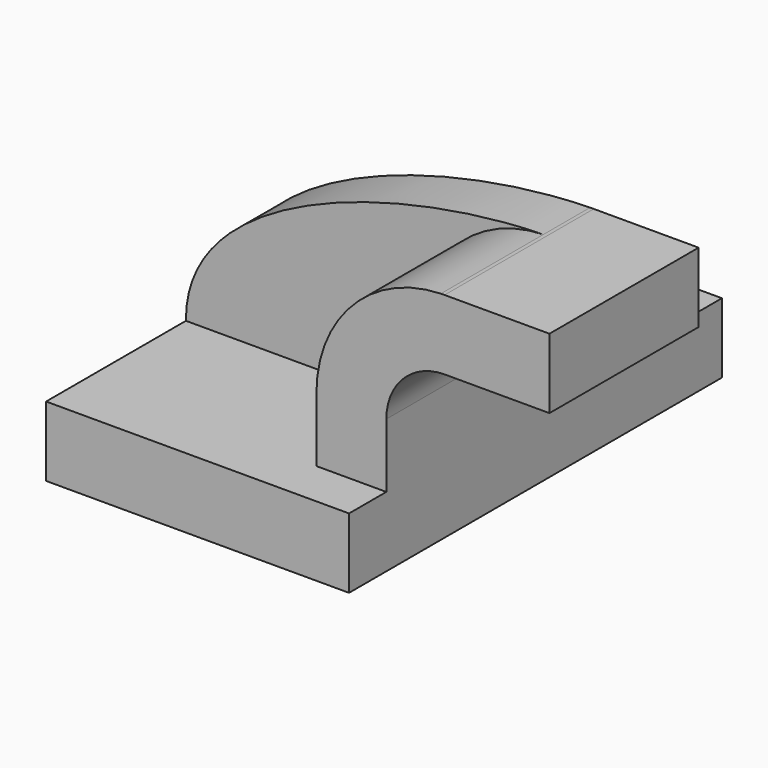
from build123d import *

# Parameters (mm, degrees)
F1_DEPTH = 63.5
F0_W     = 25.4
F0_H     = 19.0500033191
F2_DEPTH = 50.8
F3_DEPTH = 15.875


# Not quite as in the source:
# - ends of sketch curves that miss each other by under 0.0002 mm in the source are joined


with BuildPart() as f1:
    # F0 (on Front) → F1 (new body, symmetric)
    with BuildSketch(Plane.XZ):
        Polygon((-41.275, 9.525), (-41.275, -9.525), (41.275, -9.525), (41.275, 9.525), (22.225, 9.525), align=None)
    extrude(amount=F1_DEPTH, both=True)

    # F0 (on Front) → F2 (join)
    with BuildSketch(Plane.XZ):
        with BuildLine():
            Line((22.225, 9.525), (41.275, 9.525))
            Line((41.275, 9.525), (41.275, 27.0002))
            ThreePointArc((41.275, 27.0002), (45.9246798487, 38.2255201513), (57.15, 42.8752))
            Line((57.15, 42.8752), (60.325, 42.8751966809))
            Line((60.325, 42.8751966809), (60.325, 61.9252))
            Line((60.325, 61.9252), (57.15, 61.9252))
            add(Edge.make_bspline(
                [(56.1392549791, 61.9105712312), (56.4777228602, 61.916713038), (56.8146554612, 61.9215892093), (57.15, 61.9252)],
                knots=[110.5401994714, 110.5401994714, 110.5401994714, 110.5401994714, 111.5045361635, 111.5045361635, 111.5045361635, 111.5045361635], degree=3))
            ThreePointArc((56.1392549791, 61.9105712312), (32.0994920725, 51.3359284167), (22.225, 27.0002))
            Line((22.225, 27.0002), (22.225, 9.525))
        make_face()
        with Locations((73.025, 52.4001983404)):
            Rectangle(F0_W, F0_H)
    extrude(amount=F2_DEPTH)

    # F0 (on Front) → F3 (join)
    with BuildSketch(Plane.XZ):
        with BuildLine():
            add(Edge.make_bspline(
                [(-41.275, 9.525), (-41.6296994967, 43.8725434099), (17.341283892, 61.2065468529), (56.1392549791, 61.9105712312)],
                knots=[0, 0, 0, 0, 110.5401994714, 110.5401994714, 110.5401994714, 110.5401994714], degree=3))
            Line((-41.275, 9.525), (22.225, 9.525))
            Line((22.225, 9.525), (22.225, 27.0002))
            ThreePointArc((22.225, 27.0002), (32.0994920725, 51.3359284167), (56.1392549791, 61.9105712312))
        make_face()
    extrude(amount=F3_DEPTH)


solid = f1.part
